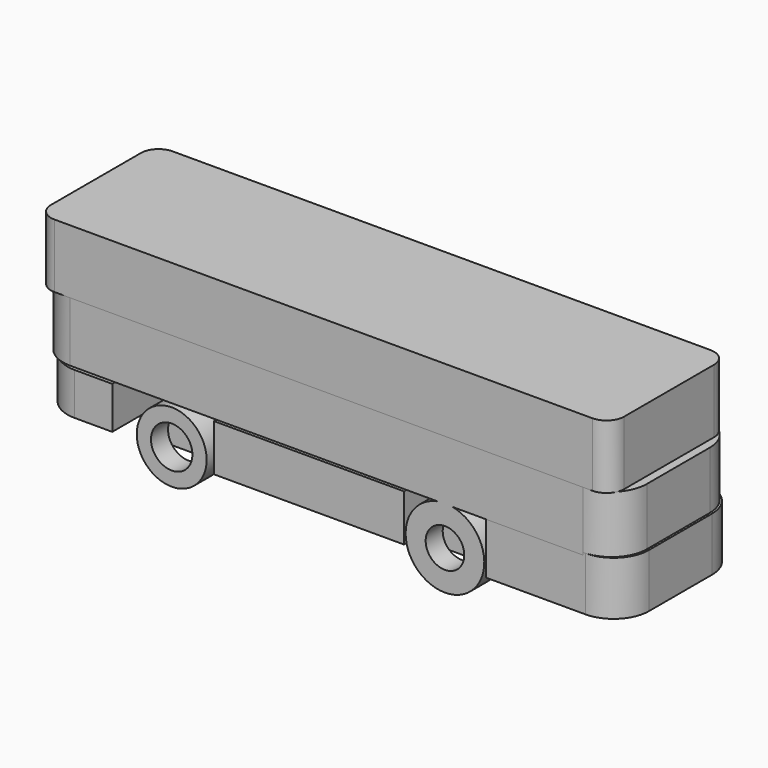
from build123d import *

# Parameters (mm, degrees)
F0_W         = 83.9661955833
F0_H         = 8.6036846042
F2_DEPTH     = 10.7490709051
F1_W         = 27.3526310921
F1_H         = 6.7362785339
F1_W_2       = 19.4012820721
F1_H_2       = 7.7336356044
F1_W_3       = 10.4926526546
F1_H_3       = 6.0765519738
F4_R         = 5.08
F5_R         = 5.08
F3_R         = 5.6577404846
F3_R_2       = 2.7776319259
F6_DEPTH     = 3.0659101903
F3_R_3       = 5.0275038218
F3_R_4       = 2.978926648
F7_R         = 5.08
F8_R         = 5.08
F10_W        = 9.2010200024
F10_H        = 12.6288309693
F10_W_2      = 7.8585743904
F10_H_2      = 13.5450959206
F11_DEPTH    = 16.8703179806
F20_W        = 21.2450809777
F20_H        = 9.1825369745
F21_DEPTH    = 49.1361897439
F22_T1_DEPTH = 15.5325369745
F23_DEPTH    = 33.3159770817
F24_R        = 2.54


# Not quite as in the source:
# - a fillet or chamfer that OpenCascade refuses, or shapes differently, is made with other operations: its cross-section is extruded or revolved along the edge and cut away or added
# - a feature names something its author has since deleted; it is built from what else it names
# - the program builds the solid bodies; features that only make, move or delete a surface that nothing else refers to are left out


with BuildPart() as f2:
    # F0 (on Front) → F2 (new body, symmetric)
    with BuildSketch(Plane.XZ):
        with Locations((8.359849453, -4.3018423021)):
            Rectangle(F0_W, F0_H)
    extrude(amount=F2_DEPTH, both=True)

    # F4
    f4_edges = [f2.edges().sort_by_distance(p)[0] for p in [
        (50.342947, 10.749071, -4.301842),
        (50.342947, -10.749071, -4.301842),
    ]]
    fillet(f4_edges, radius=F4_R)

    # F3 (on face) → F6 (join)
    with BuildSketch(Plane(origin=(0, 10.7490709051, 0), x_dir=(-1, 0, 0), z_dir=(0, 1, 0))):
        with Locations((-25.3703502001, -14.1578875482)):
            Circle(F3_R)
        with Locations((-25.3703502001, -14.1578875482)):
            Circle(F3_R_2, mode=Mode.SUBTRACT)
    extrude(amount=-F6_DEPTH)

    # F7
    f7_edges = [f2.edges().sort_by_distance(p)[0] for p in [
        (-33.623248, -10.749071, -4.301842),
        (-33.623248, 10.749071, -4.301842),
    ]]
    fillet(f7_edges, radius=F7_R)

    # F9: F2, F6 across plane


with BuildPart() as f2b:
    # F1 (on Front) → F2, piece 2 (new body, symmetric)
    with BuildSketch(Plane.XZ):
        with Locations((5.8154165745, -12.272760272)):
            Rectangle(F1_W, F1_H)
    extrude(amount=F2_DEPTH, both=True)


with BuildPart() as f2c:
    # F1 (on Front) → F2, piece 3 (new body, symmetric)
    with BuildSketch(Plane.XZ):
        with Locations((40.9603565931, -12.1280737221)):
            Rectangle(F1_W_2, F1_H_2)
    extrude(amount=F2_DEPTH, both=True)

    # F5
    f5_edges = [f2c.edges().sort_by_distance(p)[0] for p in [
        (50.660998, 10.749071, -12.128074),
        (50.660998, -10.749071, -12.128074),
    ]]
    fillet(f5_edges, radius=F5_R)


with BuildPart() as f2d:
    # F1 (on Front) → F2, piece 4 (new body, symmetric)
    with BuildSketch(Plane.XZ):
        with Locations((-27.7377068996, -11.981267482)):
            Rectangle(F1_W_3, F1_H_3)
    extrude(amount=F2_DEPTH, both=True)

    # F8
    f8_edges = [f2d.edges().sort_by_distance(p)[0] for p in [
        (-32.984033, 10.749071, -11.981267),
        (-32.984033, -10.749071, -11.981267),
    ]]
    fillet(f8_edges, radius=F8_R)


with BuildPart() as f6:
    # F3 (on face) → F6, piece 2 (new body)
    with BuildSketch(Plane(origin=(0, 10.7490709051, 0), x_dir=(-1, 0, 0), z_dir=(0, 1, 0))):
        with Locations((13.9378588647, -14.1578875482)):
            Circle(F3_R_3)
        with Locations((13.9378588647, -14.1578875482)):
            Circle(F3_R_4, mode=Mode.SUBTRACT)
    extrude(amount=-F6_DEPTH)


with BuildPart() as f2_1:
    add(f2.part)
    add(f2.part.mirror(Plane.XZ))
    add(f6.part.mirror(Plane.XZ))

    # F10 (on Top) → F11 (join)
    with BuildSketch(Plane.XY):
        with Locations((-13.9741003513, 0)):
            Rectangle(F10_W, F10_H)
        with Locations((25.6728827953, 0)):
            Rectangle(F10_W_2, F10_H_2)
    extrude(amount=-F11_DEPTH)

    # F20 (on Right) → F21 (join)
    with BuildSketch(Plane.YZ):
        with Locations((-0.1486409456, 4.5912684873)):
            Rectangle(F20_W, F20_H)
    extrude(amount=F21_DEPTH)

    # F22: fillet of radius 2.54 on 2 edges, made by hand

    # F22_s2 → F22_t1 (cut)
    with BuildSketch(Plane.XY):
        with BuildLine():
            ThreePointArc((49.1361897439, -8.2311814344), (48.3922409681, -10.0272326586), (46.5961897439, -10.7711814344))
            Line((46.5961897439, -10.7711814344), (49.1361897439, -10.7711814344))
            Line((49.1361897439, -10.7711814344), (49.1361897439, -8.2311814344))
        make_face()
        with BuildLine():
            ThreePointArc((46.5961897439, 10.4738995433), (48.3922409681, 9.7299507675), (49.1361897439, 7.9338995433))
            Line((49.1361897439, 7.9338995433), (49.1361897439, 10.4738995433))
            Line((49.1361897439, 10.4738995433), (46.5961897439, 10.4738995433))
        make_face()
    extrude(amount=F22_T1_DEPTH, mode=Mode.SUBTRACT)

    # F23 (add): a face of the model
    f23_faces = [f2_1.faces().sort_by_distance(p)[0] for p in [
        (0, -0.1486409456, 4.5912684873),
    ]]
    extrude(f23_faces, amount=F23_DEPTH)

    # F24
    f24_edges = [f2_1.edges().sort_by_distance(p)[0] for p in [
        (-33.315977, 10.4739, 4.591268),
        (-33.315977, -10.771181, 4.591268),
    ]]
    fillet(f24_edges, radius=F24_R)


solid = Compound([f2b.part, f2c.part, f2d.part, f6.part, f2_1.part])
